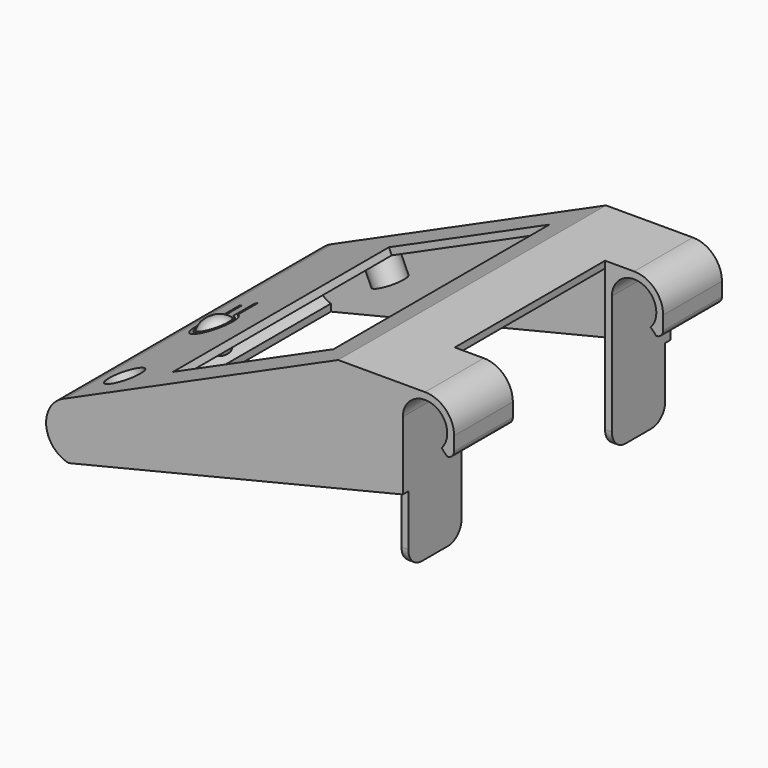
from build123d import *

# Parameters (mm, degrees)
F1_DEPTH  = 49
F2_W      = 51.5
F2_H      = 79
F3_DEPTH  = 2
F2_R      = 1.5
F2_R_2    = 4.5
F4_DEPTH  = 7.3
F6_DEPTH  = 2
F8_DEPTH  = 2
F2_R_3    = 5
F9_DEPTH  = 2
F11_DEPTH = 2
F12_W     = 8.5
F12_H     = 55
F13_DEPTH = 40
F14_R     = 1.99999
F15_W     = 2
F15_H     = 19.5
F16_DEPTH = 20
F17_W     = 2
F17_H     = 19.5
F18_DEPTH = 20
F19_R     = 5
F20_DEPTH = 2
F21_R     = 2.5
F22_DEPTH = 7.5
F21_R_2   = 4.5
F23_DEPTH = 2
F25_R     = 2


# Not quite as in the source:
# - a fillet or chamfer that OpenCascade refuses, or shapes differently, is made with other operations: its cross-section is extruded or revolved along the edge and cut away or added
# - a fillet or chamfer is up to 0.001 mm smaller than in the source, because OpenCascade refuses the exact size
# - a feature names something its author has since deleted; it is built from what else it names


with BuildPart() as f1:
    # F0 (on Front) → F1 (new body, symmetric)
    with BuildSketch(Plane.XZ):
        with BuildLine():
            Line((-25, 6.5), (-8.5, 6.5))
            Line((-8.5, 6.5), (-8.5, 0))
            Line((-8.5, 0), (-8.5, -20))
            Line((-8.5, -20), (-6.5, -20))
            Line((-6.5, -20), (-6.5, 0))
            ThreePointArc((-6.5, 0), (2.3181097502, 6.072591472), (4.8465745188, -4.3313641539))
            Line((4.8465745188, -4.3313641539), (6.5, -6))
            Line((6.5, -6), (8.5, -6))
            Line((8.5, -6), (8.5, 0))
            ThreePointArc((8.5, 0), (6.0104076401, 6.0104076401), (0, 8.5))
            Line((0, 8.5), (-25.4288327804, 8.5))
            Line((-25.4288327804, 8.5), (-105.428633061, -27.4597649849))
            Line((-105.428633061, -27.4597649849), (-106.3520655314, -27.8748462039))
            ThreePointArc((-106.3520655314, -27.8748462039), (-110.8598066956, -36.4968976222), (-104.3520655314, -43.7293803221))
            Line((-104.3520655314, -43.7293803221), (-104.3520655314, -42.85))
            Line((-104.3520655314, -42.85), (-104.3520655314, -41.6571435378))
            ThreePointArc((-104.3520655314, -41.6571435378), (-108.9268429391, -35.4298576938), (-104.3520655314, -29.2025718498))
            Line((-104.3520655314, -29.2025718498), (-104.3520655314, -29.1686093911))
            Line((-104.3520655314, -29.1686093911), (-25, 6.5))
        make_face()
    extrude(amount=F1_DEPTH, both=True)

    # F2 (on face) → F3 (cut)
    with BuildSketch(Plane(origin=(-6.6328046362, 0, 14.75602097), x_dir=(0.9120927073, 0, 0.409984016), z_dir=(0.409984016, 0, -0.9120927073))):
        with Locations((-55.3874215775, -0.1)):
            Rectangle(F2_W, F2_H)
    extrude(amount=-F3_DEPTH, mode=Mode.SUBTRACT)

    # F2 (on face) → F4 (join)
    with BuildSketch(Plane(origin=(-6.6328046362, 0, 14.75602097), x_dir=(0.9120927073, 0, 0.409984016), z_dir=(0.409984016, 0, -0.9120927073))):
        with BuildLine():
            Line((-20.1374215775, 40.7130369812), (-20.1374215775, 47.9869630188))
            ThreePointArc((-20.1374215775, 47.9869630188), (-27.2874215775, 44.35), (-20.1374215775, 40.7130369812))
        make_face()
        with Locations((-22.7874215775, 44.35)):
            Circle(F2_R, mode=Mode.SUBTRACT)
        with BuildLine():
            Line((-20.1374215775, -47.5869630188), (-20.1374215775, -40.3130369812))
            ThreePointArc((-20.1374215775, -40.3130369812), (-27.2874215775, -43.95), (-20.1374215775, -47.5869630188))
        make_face()
        with Locations((-22.7874215775, -43.95)):
            Circle(F2_R, mode=Mode.SUBTRACT)
        with Locations((-88.7874215775, -43.95)):
            Circle(F2_R_2)
        with Locations((-88.7874215775, -43.95)):
            Circle(F2_R, mode=Mode.SUBTRACT)
        with Locations((-88.7874215775, 44.35)):
            Circle(F2_R_2)
        with Locations((-88.7874215775, 44.35)):
            Circle(F2_R, mode=Mode.SUBTRACT)
    extrude(amount=F4_DEPTH)

    # F5 (on face) → F6 (join)
    with BuildSketch(Plane.XZ.offset(49)):
        with BuildLine():
            Line((-104.3520655314, -43.7293803221), (-6.5, -20))
            Line((-6.5, -20), (-8.5, -20))
            Line((-8.5, -20), (-8.5, 6.5))
            Line((-8.5, 6.5), (-25, 6.5))
            Line((-25, 6.5), (-104.3520655314, -29.1686093911))
            Line((-104.3520655314, -29.1686093911), (-104.3520655314, -29.2025718498))
            ThreePointArc((-104.3520655314, -29.2025718498), (-108.9268429391, -35.4298576938), (-104.3520655314, -41.6571435378))
            Line((-104.3520655314, -41.6571435378), (-104.3520655314, -43.7293803221))
        make_face()
    extrude(amount=-F6_DEPTH)

    # F7 (on face) → F8 (join)
    with BuildSketch(Plane(origin=(0, 49, 0), x_dir=(-1, 0, 0), z_dir=(0, 1, 0))):
        with BuildLine():
            Line((8.5, -20), (6.5, -20))
            Line((6.5, -20), (104.3520655314, -43.7293803221))
            Line((104.3520655314, -43.7293803221), (104.3520655314, -41.6571435378))
            ThreePointArc((104.3520655314, -41.6571435378), (108.9268429391, -35.4298576938), (104.3520655314, -29.2025718498))
            Line((104.3520655314, -29.2025718498), (104.3520655314, -29.1686093911))
            Line((104.3520655314, -29.1686093911), (25, 6.5))
            Line((25, 6.5), (8.5, 6.5))
            Line((8.5, 6.5), (8.5, -20))
        make_face()
    extrude(amount=-F8_DEPTH)

    # F2 (on face) → F9 (cut)
    with BuildSketch(Plane(origin=(-6.6328046362, 0, 14.75602097), x_dir=(0.9120927073, 0, 0.409984016), z_dir=(0.409984016, 0, -0.9120927073))):
        with Locations((-98.7513456427, 37)):
            Circle(F2_R_3)
    extrude(amount=-F9_DEPTH, mode=Mode.SUBTRACT)

    # F10 (on face) → F11 (cut)
    with BuildSketch(Plane(origin=(0, 49, 0), x_dir=(-1, 0, 0), z_dir=(0, 1, 0))):
        Polygon((63.2235160953, -24.4957862935), (39.5091057066, -13.8362018777), (38.0741616506, -17.0285263531), (61.7885720393, -27.6881107689), align=None)
    extrude(amount=-F11_DEPTH, mode=Mode.SUBTRACT)

    # F12 (on face) → F13 (cut)
    with BuildSketch(Plane.XY.offset(8.5)):
        with Locations((4.25, 0)):
            Rectangle(F12_W, F12_H)
        with Locations((-4.25, 0)):
            Rectangle(F12_W, F12_H)
    extrude(amount=-F13_DEPTH, mode=Mode.SUBTRACT)

    # F14 (radius 2 in the source; OpenCascade refuses exactly that, so slightly less here)
    f14_edges = [f1.edges().sort_by_distance(p)[0] for p in [
        (8.5, 38.25, -6),
        (8.5, -38.25, -6),
    ]]
    fillet(f14_edges, radius=F14_R)

    # F15 (on face) → F16 (join)
    with BuildSketch(Plane(origin=(0, 0, -20), x_dir=(1, 0, 0), z_dir=(0, 0, -1))):
        with Locations((-7.5, 37.25)):
            Rectangle(F15_W, F15_H)
    extrude(amount=F16_DEPTH)

    # F17 (on face) → F18 (join)
    with BuildSketch(Plane(origin=(0, 0, -20), x_dir=(1, 0, 0), z_dir=(0, 0, -1))):
        with Locations((-7.5, -37.25)):
            Rectangle(F17_W, F17_H)
    extrude(amount=F18_DEPTH)

    # F19
    f19_edges = [f1.edges().sort_by_distance(p)[0] for p in [
        (-7.5, 47, -40),
        (-7.5, 27.5, -40),
        (-7.5, -27.5, -40),
        (-7.5, -47, -40),
    ]]
    fillet(f19_edges, radius=F19_R)

    # F2 (on face) → F20 (cut)
    with BuildSketch(Plane(origin=(-6.6328046362, 0, 14.75602097), x_dir=(0.9120927073, 0, 0.409984016), z_dir=(0.409984016, 0, -0.9120927073))):
        with BuildLine():
            ThreePointArc((-100.7513456427, -0.282575695), (-98.7513456427, 9.3), (-96.7513456427, -0.282575695))
            Line((-96.7513456427, -0.282575695), (-96.7513456427, -8.282575695))
            Line((-96.7513456427, -8.282575695), (-95.7513456427, -8.282575695))
            Line((-95.7513456427, -8.282575695), (-95.7513456427, -0.8961524227))
            ThreePointArc((-95.7513456427, -0.8961524227), (-98.7513456427, 10.3), (-101.7513456427, -0.8961524227))
            Line((-101.7513456427, -0.8961524227), (-101.7513456427, -8.282575695))
            Line((-101.7513456427, -8.282575695), (-100.7513456427, -8.282575695))
            Line((-100.7513456427, -8.282575695), (-100.7513456427, -0.282575695))
        make_face()
    extrude(amount=-F20_DEPTH, mode=Mode.SUBTRACT)

    # F21 (on face) → F22 (join)
    with BuildSketch(Plane(origin=(-7.4527726682, 0, 16.5802063845), x_dir=(0.9120927073, 0, 0.409984016), z_dir=(-0.409984016, 0, 0.9120927073))):
        with Locations((-98.7513456427, -4.3)):
            Circle(F21_R)
    extrude(amount=-F22_DEPTH)

    # F21 (on face) → F23 (join)
    with BuildSketch(Plane(origin=(-7.4527726682, 0, 16.5802063845), x_dir=(0.9120927073, 0, 0.409984016), z_dir=(-0.409984016, 0, 0.9120927073))):
        with Locations((-98.7513456427, -4.3)):
            Circle(F21_R_2)
        with Locations((-98.7513456427, -4.3)):
            Circle(F21_R, mode=Mode.SUBTRACT)
        with Locations((-98.7513456427, -4.3)):
            Circle(F21_R)
    extrude(amount=F23_DEPTH)

    # F24: fillet of radius 5 on 1 edges, made by hand

    # F24_s1 → F24_t2 (revolve, cut)
    with BuildSketch(Plane.XZ.offset(4.3)):
        with BuildLine():
            ThreePointArc((-93.4187376781, -22.0613388145), (-95.6311594228, -21.4417982804), (-97.8870765391, -21.877089464))
            Line((-97.8870765391, -21.877089464), (-94.2387057101, -20.2371534))
            Line((-94.2387057101, -20.2371534), (-93.4187376781, -22.0613388145))
        make_face()
    revolve(axis=Axis((-98.3431228928, -4.3, -22.082081472), (-0.409984016, 0, 0.9120927073)), mode=Mode.SUBTRACT)

    # F25
    f25_edges = [f1.edges().sort_by_distance(p)[0] for p in [
        (-96.728507, -4.3, -31.771922),
    ]]
    fillet(f25_edges, radius=F25_R)


solid = f1.part
